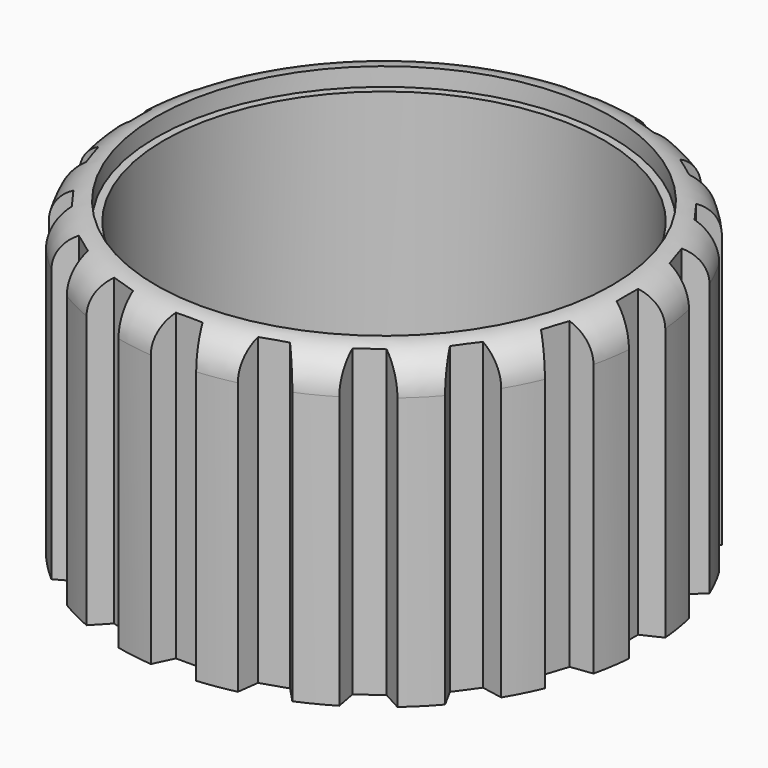
from build123d import *

# Parameters (mm, degrees)
F3_DEPTH        = 40
F3_COPIES_COUNT = 20


# Not quite as in the source:
# - a pattern or mirror of a feature is missing from the dataset's text; its kind, count and spacing are read off the source's solid


with BuildPart() as f1:
    # F0 (on Front) → F1 (revolve)
    with BuildSketch(Plane.XZ):
        with BuildLine():
            ThreePointArc((-25.9039036185, 35), (-28.8002811462, 33.8002811462), (-30, 30.9039036185))
            Line((-30, 30.9039036185), (-30, 0))
            Line((-30, 0), (0, 0))
            Line((0, 0), (0, 2.9404360056))
            Line((0, 2.9404360056), (-25, 2.9404360056))
            Line((-25, 2.9404360056), (-25, 32.9404360056))
            Line((-25, 32.9404360056), (-25.8917759359, 32.9404360056))
            Line((-25.8917759359, 32.9404360056), (-25.9039036185, 35))
        make_face()
    revolve(axis=Axis((0, 0, 1.4702180028), (0, 0, -1)))

    # F2 (on Top) → F3 (cut)
    with BuildSketch(Plane.XY):
        Polygon((3.2103396952, 31.2208756804), (-3.2103396952, 31.2208756804), (-1.5207296237, 27.653047815), (0, 27.653047815), (1.5207296237, 27.653047815), align=None)
    f3 = extrude(amount=F3_DEPTH, mode=Mode.SUBTRACT)

    # F3_copies: F3 ×20 about axis
    f3_copies_axis = Axis((0, 0, 0), (0, 0, 1))
    for i in range(1, F3_COPIES_COUNT):
        add(f3.rotate(f3_copies_axis, i * 360 / F3_COPIES_COUNT), mode=Mode.SUBTRACT)


solid = f1.part
